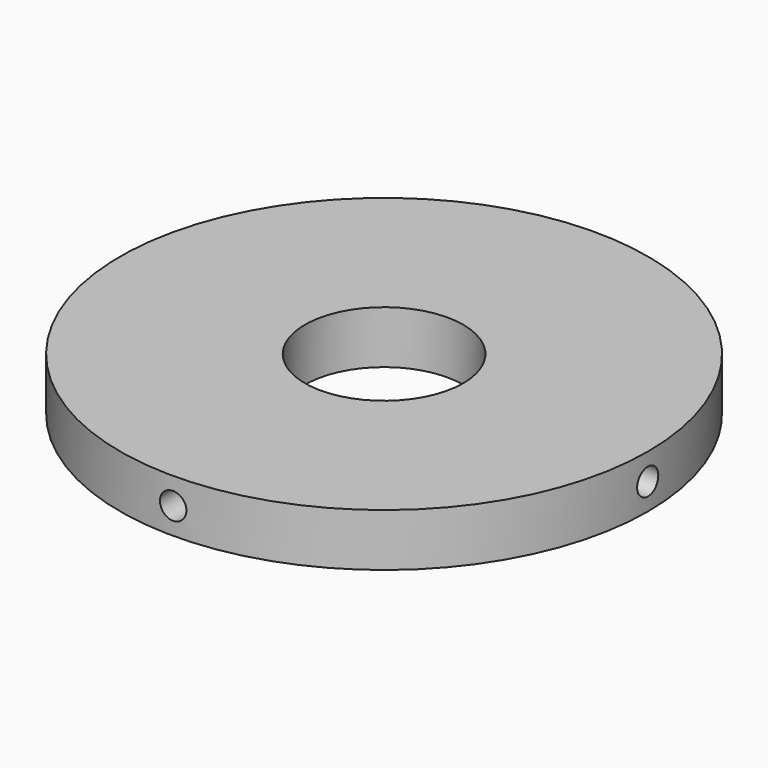
from build123d import *

# Parameters (mm, degrees)
F0_R      = 20
F0_R_2    = 6
F1_DEPTH  = 2
F4_D      = 2
F4_DEPTH  = 3
F4_TIP    = 0.600860619
F7_D      = 2
F7_DEPTH  = 3
F7_TIP    = 0.600860619
F10_D     = 2
F10_DEPTH = 3
F10_TIP   = 0.600860619
F13_D     = 2
F13_DEPTH = 3
F13_TIP   = 0.600860619


with BuildPart() as f1:
    # F0 (on Top) → F1 (new body, symmetric)
    with BuildSketch(Plane.XY):
        Circle(F0_R)
        Circle(F0_R_2, mode=Mode.SUBTRACT)
    extrude(amount=F1_DEPTH, both=True)

    # F4 (one way)
    with BuildSketch(Plane.YZ.offset(20)):
        with Locations((0, 0)):
            Circle(F4_D / 2)
    extrude(amount=-F4_DEPTH, mode=Mode.SUBTRACT)
    with Locations(Plane.YZ.offset(20)):
        with Locations((0, 0)):
            with Locations((0, 0, -(F4_DEPTH + F4_TIP / 2))):  # 118° drill point
                Cone(0, F4_D / 2, F4_TIP, mode=Mode.SUBTRACT)

    # F7 (one way)
    with BuildSketch(Plane(origin=(-20, 0, 0), x_dir=(0, 1, 0), z_dir=(-1, 0, 0))):
        with Locations((0, 0)):
            Circle(F7_D / 2)
    extrude(amount=-F7_DEPTH, mode=Mode.SUBTRACT)
    with Locations(Plane(origin=(-20, 0, 0), x_dir=(0, 1, 0), z_dir=(-1, 0, 0))):
        with Locations((0, 0)):
            with Locations((0, 0, -(F7_DEPTH + F7_TIP / 2))):  # 118° drill point
                Cone(0, F7_D / 2, F7_TIP, mode=Mode.SUBTRACT)

    # F10 (one way)
    with BuildSketch(Plane.XZ.offset(20)):
        with Locations((0, 0)):
            Circle(F10_D / 2)
    extrude(amount=-F10_DEPTH, mode=Mode.SUBTRACT)
    with Locations(Plane.XZ.offset(20)):
        with Locations((0, 0)):
            with Locations((0, 0, -(F10_DEPTH + F10_TIP / 2))):  # 118° drill point
                Cone(0, F10_D / 2, F10_TIP, mode=Mode.SUBTRACT)

    # F13 (one way)
    with BuildSketch(Plane(origin=(0, 20, 0), x_dir=(1, 0, 0), z_dir=(0, 1, 0))):
        with Locations((0, 0)):
            Circle(F13_D / 2)
    extrude(amount=-F13_DEPTH, mode=Mode.SUBTRACT)
    with Locations(Plane(origin=(0, 20, 0), x_dir=(1, 0, 0), z_dir=(0, 1, 0))):
        with Locations((0, 0)):
            with Locations((0, 0, -(F13_DEPTH + F13_TIP / 2))):  # 118° drill point
                Cone(0, F13_D / 2, F13_TIP, mode=Mode.SUBTRACT)


solid = f1.part
